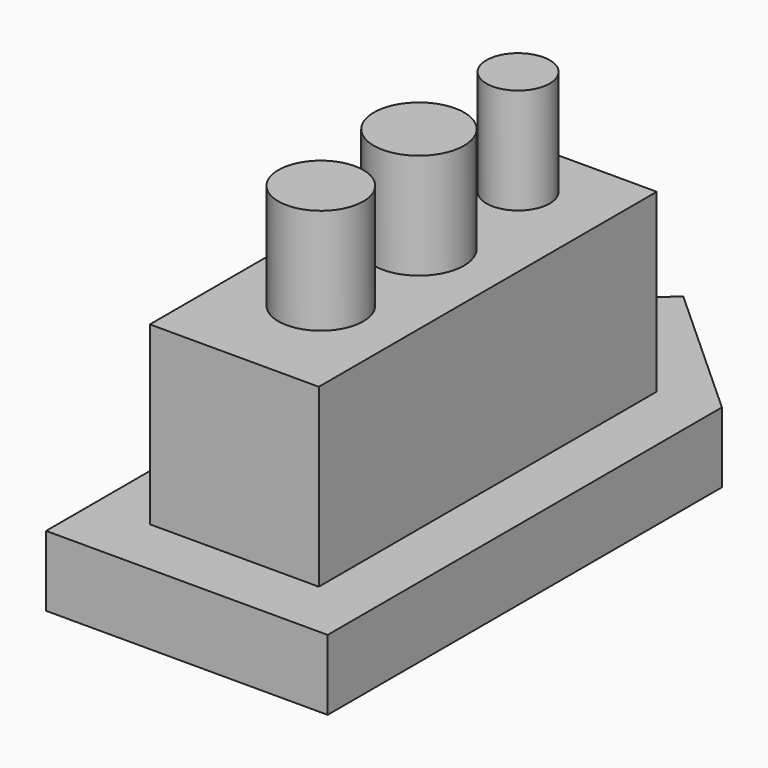
from build123d import *

# Parameters (mm, degrees)
F1_DEPTH     = 10
F2_W         = 24
F2_H         = 60
F4_DEPTH     = 25
F5_R         = 4.5
F6_DEPTH     = 15
F5_R_2       = 6.4027170917
F5_R_3       = 6.0335625596
F7_TEXT_SIZE = 12.9833662262
F8_DEPTH     = 15


# Not quite as in the source:
# - Text() gives the source's letters only with a copy of the font that has no kerning and outlines rounded to 1/6400 em; it was checked with that copy


with BuildPart() as f1:
    # F0 (on Top) → F1 (new body)
    with BuildSketch(Plane.XY):
        Polygon((0, 51.1274002164), (-20, 32.9890430691), (-20, -37.0109569309), (20, -37.0109569309), (20, 32.9890430691), align=None)
    extrude(amount=F1_DEPTH)

    # F2 (on face) → F4 (join)
    with BuildSketch(Plane.XY.offset(10)):
        with Locations((0, 1.4163665473)):
            Rectangle(F2_W, F2_H)
    extrude(amount=F4_DEPTH)

    # F7 (on face) → F8 (cut)
    with BuildSketch(Plane(origin=(-12, 0, 0), x_dir=(0, -1, 0), z_dir=(-1, 0, 0))):
        with Locations((-14.6142147302, 18.8376810402)):
            Text('sabic', F7_TEXT_SIZE, font='Open Sans', font_style=FontStyle.BOLD, text_align=(TextAlign.LEFT, TextAlign.BOTTOM))
    extrude(amount=-F8_DEPTH, mode=Mode.SUBTRACT)


with BuildPart() as f6:
    # F5 (on face) → F6 (new body)
    with BuildSketch(Plane.XY.offset(35)):
        with Locations((0, 21.7950149111)):
            Circle(F5_R)
    extrude(amount=F6_DEPTH)


with BuildPart() as f6b:
    # F5 (on face) → F6, piece 2 (new body)
    with BuildSketch(Plane.XY.offset(35)):
        with Locations((0, 4.1965556578)):
            Circle(F5_R_2)
    extrude(amount=F6_DEPTH)


with BuildPart() as f6c:
    # F5 (on face) → F6, piece 3 (new body)
    with BuildSketch(Plane.XY.offset(35)):
        with Locations((0, -13.2228294387)):
            Circle(F5_R_3)
    extrude(amount=F6_DEPTH)


solid = Compound([f1.part, f6.part, f6b.part, f6c.part])
